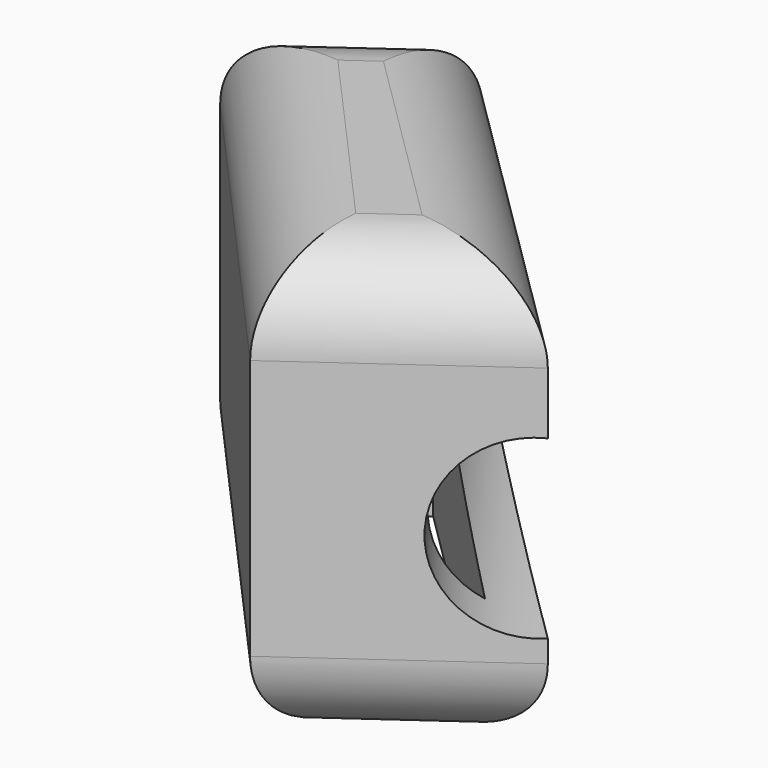
from build123d import *

# Parameters (mm, degrees)
F1_DEPTH    = 25.4
F2_R        = 5.08
F3_T        = -2.54
F4_T1_DEPTH = 50.8
F4_T3_DEPTH = 39.0278032796
F4_T5_DEPTH = 51.0230548821
F4_T7_DEPTH = 37.4321438382
F6_DEPTH    = 105.664


# Not quite as in the source:
# - a fillet or chamfer that OpenCascade refuses, or shapes differently, is made with other operations: its cross-section is extruded or revolved along the edge and cut away or added


with BuildPart() as f1:
    # F0 (on Top) → F1 (new body)
    with BuildSketch(Plane.XY):
        Polygon((-0.8999820115, 8.1055370808), (-10.6966300514, 1.1199682045), (6.2161790492, -17.8304114309), (17.312023155, -9.9184416504), align=None)
    extrude(amount=F1_DEPTH)

    # F2
    f2_edges = [f1.edges().sort_by_distance(p)[0] for p in [
        (8.206021, -0.906452, 25.4),
        (11.764101, -13.874427, 25.4),
        (-2.240226, -8.355222, 25.4),
        (-5.798306, 4.612753, 25.4),
    ]]
    fillet(f2_edges, radius=F2_R)

    # F3
    f3_openings = [f1.faces().sort_by_distance(p)[0] for p in [
        (3.164917, -4.822441, 0),
    ]]
    offset(amount=F3_T, openings=f3_openings)

    # F4: fillet of radius 5.08 on 4 edges, made by hand

    # F4_s2 → F4_t1 (cut)
    with BuildSketch(Plane(origin=(-13.7553254463, 15.4124981643, 0), x_dir=(0, 0, 1), z_dir=(0.665858626, -0.7460779384, 0))):
        with BuildLine():
            ThreePointArc((5.08, 7.2347792067), (1.4878975516, 5.7468816552), (0, 2.1547792067))
            Line((0, 2.1547792067), (0, 7.2347792067))
            Line((0, 7.2347792067), (5.08, 7.2347792067))
        make_face()
    extrude(amount=F4_T1_DEPTH, mode=Mode.SUBTRACT)

    # F4_s4 → F4_t3 (cut)
    with BuildSketch(Plane(origin=(-14.6481007776, -10.4449314165, 0), x_dir=(0, 0, 1), z_dir=(0.8142063602, 0.5805755791, 0))):
        with BuildLine():
            ThreePointArc((5.08, 18.1265961431), (1.4878975516, 16.6386985916), (0, 13.0465961431))
            Line((0, 13.0465961431), (0, 18.1265961431))
            Line((0, 18.1265961431), (5.08, 18.1265961431))
        make_face()
    extrude(amount=F4_T3_DEPTH, mode=Mode.SUBTRACT)

    # F4_s6 → F4_t5 (cut)
    with BuildSketch(Plane(origin=(22.7315266592, -22.496839271, 0), x_dir=(0, 0, 1), z_dir=(-0.7107663489, 0.7034281749, 0))):
        with BuildLine():
            ThreePointArc((5.08, 5.1280702931), (1.4878975516, 3.6401727415), (0, 0.0480702931))
            Line((0, 0.0480702931), (0, 5.1280702931))
            Line((0, 5.1280702931), (5.08, 5.1280702931))
        make_face()
    extrude(amount=F4_T5_DEPTH, mode=Mode.SUBTRACT)

    # F4_s8 → F4_t7 (cut)
    with BuildSketch(Plane(origin=(13.575348792, 9.6799980584, 0), x_dir=(0, 0, 1), z_dir=(-0.8142063602, -0.5805755791, 0))):
        with BuildLine():
            ThreePointArc((5.08, 7.1220874215), (1.4878975516, 5.6341898699), (0, 2.0420874215))
            Line((0, 2.0420874215), (0, 7.1220874215))
            Line((0, 7.1220874215), (5.08, 7.1220874215))
        make_face()
    extrude(amount=F4_T7_DEPTH, mode=Mode.SUBTRACT)

    # F5 (on face) → F6 (cut)
    with BuildSketch(Plane(origin=(10.5238590523, -14.7587898685, 0), x_dir=(0.8142063602, 0.5805755791, 0), z_dir=(0.5805755791, -0.8142063602, 0))):
        with BuildLine():
            Line((8.3371543562, 6.3802872405), (8.3371543562, 16.698849146))
            ThreePointArc((8.3371543562, 16.698849146), (2.6890388134, 11.5395681933), (8.3371543562, 6.3802872405))
        make_face()
        with BuildLine():
            ThreePointArc((8.3371543562, 6.3802872405), (11.6943719949, 8.0457081644), (13.0499085036, 11.5395681933))
            ThreePointArc((13.0499085036, 11.5395681933), (11.6943719949, 15.0334282221), (8.3371543562, 16.698849146))
            Line((8.3371543562, 16.698849146), (8.3371543562, 6.3802872405))
        make_face()
    extrude(amount=-F6_DEPTH, mode=Mode.SUBTRACT)


solid = f1.part
